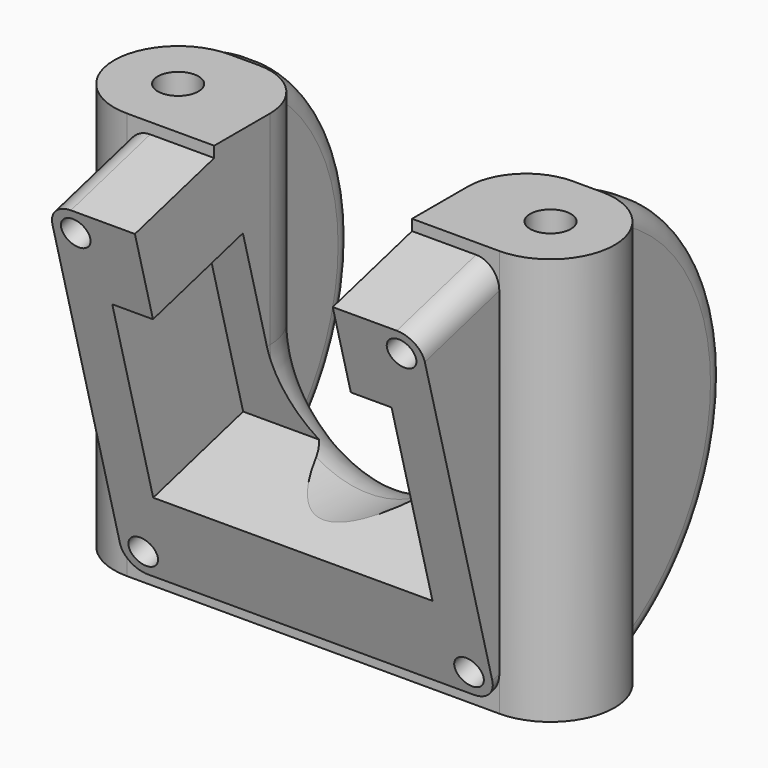
from build123d import *

# Parameters (mm, degrees)
F0_R           = 1.75
F1_DEPTH       = 35
F3_DEPTH       = 11.001
F6_REACH       = 64.9396846637
F8_DEPTH       = 25
F9_R           = 1.25
F10_DEPTH      = 4.2
F12_DEPTH      = 10
F14_DEPTH      = 2
F14_DEPTH_BACK = 2
F16_R          = 1.7
F17_T1_DEPTH   = 30
F17_T4_ANGLE   = 180


# Not quite as in the source:
# - a fillet or chamfer that OpenCascade refuses, or shapes differently, is made with other operations: its cross-section is extruded or revolved along the edge and cut away or added
# - a feature of the source that left no trace in its solid (it failed there, or was rolled back) is left out


with BuildPart() as f1:
    # F0 (on Top) → F1 (new body)
    with BuildSketch(Plane.XY):
        with BuildLine():
            Line((16, 5.5), (-16, 5.5))
            ThreePointArc((-16, 5.5), (-21.5, 0), (-16, -5.5))
            Line((-16, -5.5), (16, -5.5))
            ThreePointArc((16, -5.5), (21.5, 0), (16, 5.5))
        make_face()
        with Locations((-16, 0)):
            Circle(F0_R, mode=Mode.SUBTRACT)
        with Locations((16, 0)):
            Circle(F0_R, mode=Mode.SUBTRACT)
    extrude(amount=F1_DEPTH)

    # F2 (on face) → F3 (cut, through all)
    with BuildSketch(Plane.XZ.offset(5.5)):
        with BuildLine():
            Line((-8.5, 35), (-8.5, 17.5))
            ThreePointArc((-8.5, 17.5), (0, 9), (8.5, 17.5))
            Line((8.5, 17.5), (8.5, 35))
            Line((8.5, 35), (-8.5, 35))
        make_face()
    extrude(amount=-F3_DEPTH, mode=Mode.SUBTRACT)

    f6_end = Plane(origin=(0, -5.5, 14.4059555713), x_dir=(0, 0, -1), z_dir=(0, -1, 0))
    # F5 (on face) → F6 (join, up to a plane its end follows)
    with BuildSketch(Plane(origin=(0, -5.1315698604, -1.375), x_dir=(-1, 0, 0), z_dir=(0, 0.9659258263, 0.2588190451))):
        with BuildLine():
            ThreePointArc((16, 32.3272067081), (15.4142135624, 33.7414202705), (14, 34.3272067081))
            Line((14, 34.3272067081), (-14, 34.3272067081))
            ThreePointArc((-14, 34.3272067081), (-15.4142135624, 33.7414202705), (-16, 32.3272067081))
            Line((-16, 32.3272067081), (-16, 4.3272067081))
            ThreePointArc((-16, 4.3272067081), (-15.4142135624, 2.9129931457), (-14, 2.3272067081))
            Line((-14, 2.3272067081), (14, 2.3272067081))
            ThreePointArc((14, 2.3272067081), (15.4142135624, 2.9129931457), (16, 4.3272067081))
            Line((16, 4.3272067081), (16, 32.3272067081))
        make_face()
    f6_long = extrude(amount=F6_REACH, mode=Mode.PRIVATE)
    add(split(f6_long, bisect_by=f6_end, keep=Keep.TOP, mode=Mode.PRIVATE))

    # F7 (on face) → F8 (cut)
    with BuildSketch(Plane(origin=(0, 5.5, 0), x_dir=(-1, 0, 0), z_dir=(0, 1, 0))):
        with BuildLine():
            Line((8.5, 35), (-8.5, 35))
            Line((-8.5, 35), (-8.5, 17.5))
            ThreePointArc((-8.5, 17.5), (0, 9), (8.5, 17.5))
            Line((8.5, 17.5), (8.5, 35))
        make_face()
    extrude(amount=-F8_DEPTH, mode=Mode.SUBTRACT)

    # F9 (on face) → F10 (cut)
    with BuildSketch(Plane(origin=(0, -5.1315698604, -1.375), x_dir=(1, 0, 0), z_dir=(0, -0.9659258263, -0.2588190451))):
        with Locations((-14, 32.3272067081)):
            Circle(F9_R)
        with Locations((14, 32.3272067081)):
            Circle(F9_R)
        with Locations((14, 4.3272067081)):
            Circle(F9_R)
        with Locations((-14, 4.3272067081)):
            Circle(F9_R)
    extrude(amount=-F10_DEPTH, mode=Mode.SUBTRACT)

    # F11 (on face) → F12 (cut)
    with BuildSketch(Plane(origin=(0, -5.1315698604, -1.375), x_dir=(1, 0, 0), z_dir=(0, -0.9659258263, -0.2588190451))):
        with BuildLine():
            Line((8.5, 19.5408379052), (8.5, 26.8272067081))
            Line((8.5, 26.8272067081), (-8.5, 26.8272067081))
            Line((-8.5, 26.8272067081), (-8.5, 19.5408379052))
            add(Edge.make_bspline(
                [(8.5, 19.5408379052), (8.5, 10.7409903718), (0, 10.7409903718), (-8.5, 10.7409903718), (-8.5, 19.5408379052)],
                knots=[4.7123889804, 4.7123889804, 4.7123889804, 6.2831853072, 6.2831853072, 7.853981634, 7.853981634, 7.853981634], degree=2, weights=[1, 0.7071067812, 1, 0.7071067812, 1]))
        make_face()
        with BuildLine():
            Line((12, 9.8272067081), (12, 26.8272067081))
            Line((12, 26.8272067081), (8.5, 26.8272067081))
            Line((8.5, 26.8272067081), (8.5, 19.5408379052))
            add(Edge.make_bspline(
                [(8.5, 19.5408379052), (8.5, 10.7409903718), (0, 10.7409903718), (-8.5, 10.7409903718), (-8.5, 19.5408379052)],
                knots=[4.7123889804, 4.7123889804, 4.7123889804, 6.2831853072, 6.2831853072, 7.853981634, 7.853981634, 7.853981634], degree=2, weights=[1, 0.7071067812, 1, 0.7071067812, 1]))
            Line((-8.5, 19.5408379052), (-8.5, 26.8272067081))
            Line((-8.5, 26.8272067081), (-12, 26.8272067081))
            Line((-12, 26.8272067081), (-12, 9.8272067081))
            Line((-12, 9.8272067081), (12, 9.8272067081))
        make_face()
    extrude(amount=-F12_DEPTH, mode=Mode.SUBTRACT)

    # F13 (on face) → F14 (join, two sides)
    with BuildSketch(Plane.YZ.offset(16)) as f14_sk:
        with BuildLine():
            ThreePointArc((5.5, 0), (16.3836762358, 17.5), (5.5, 35))
            Line((5.5, 35), (5.5, 0))
        make_face()
    extrude(amount=F14_DEPTH)
    extrude(f14_sk.sketch, amount=-F14_DEPTH_BACK)

    # F15: F1 across plane


with BuildPart() as f1_1:
    add(f1.part)
    add(f1.part.mirror(Plane.YZ))

    # F16
    f16_edges = [f1_1.edges().sort_by_distance(p)[0] for p in [
        (18, 16.383676, 17.5),
        (14, 16.383676, 17.5),
        (-14, 16.383676, 17.5),
        (-18, 16.383676, 17.5),
    ]]
    fillet(f16_edges, radius=F16_R)

    # F17: fillet of radius 5 on 3 edges, made by hand

    # F17_s2 → F17_t1 (cut)
    with BuildSketch(Plane.XY.offset(17.5)):
        with BuildLine():
            ThreePointArc((13.5, 5.5), (9.9644660941, 4.0355339059), (8.5, 0.5))
            Line((8.5, 0.5), (8.5, 5.5))
            Line((8.5, 5.5), (13.5, 5.5))
        make_face()
        with BuildLine():
            ThreePointArc((-13.5, 5.5), (-9.9644660941, 4.0355339059), (-8.5, 0.5))
            Line((-8.5, 0.5), (-8.5, 5.5))
            Line((-8.5, 5.5), (-13.5, 5.5))
        make_face()
    extrude(amount=F17_T1_DEPTH, mode=Mode.SUBTRACT)

    # F17_s3 → F17_t4 (revolve, cut)
    with BuildSketch(Plane.XY.offset(17.5)):
        with BuildLine():
            ThreePointArc((-13.5, 5.5), (-9.9644660941, 4.0355339059), (-8.5, 0.5))
            Line((-8.5, 0.5), (-8.5, 5.5))
            Line((-8.5, 5.5), (-13.5, 5.5))
        make_face()
    revolve(axis=Axis((0, 5.5, 17.5), (0, -1, 0)), revolution_arc=F17_T4_ANGLE, mode=Mode.SUBTRACT)


solid = f1_1.part
